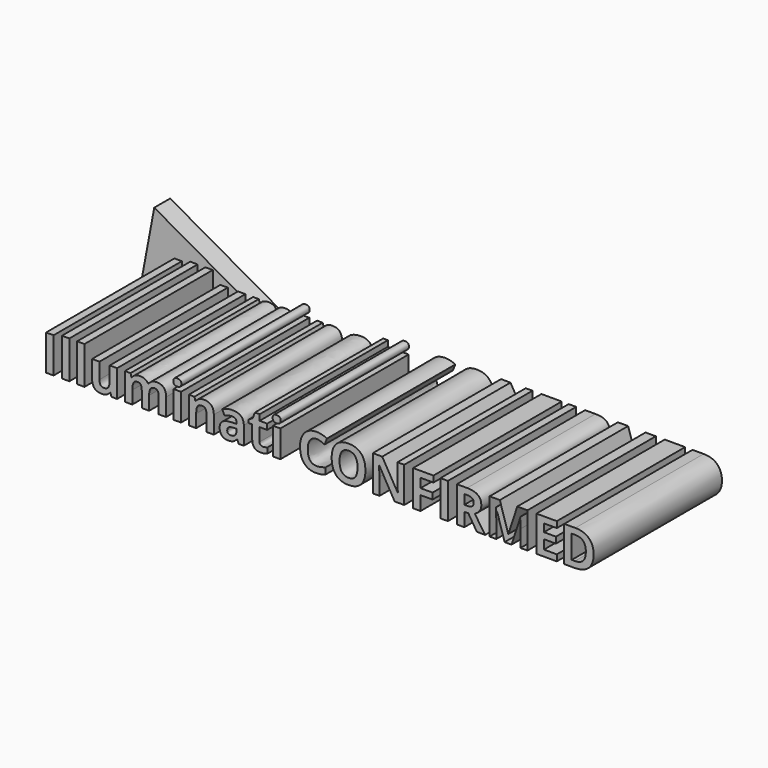
from build123d import *

# Parameters (mm, degrees)
F1_DEPTH     = 3.1
F3_TEXT_SIZE = 7.7416809897
F4_DEPTH     = 25


# Not quite as in the source:
# - Text() gives the source's letters only with a copy of the font that has no kerning and outlines rounded to 1/6400 em; it was checked with that copy


with BuildPart() as f1:
    # F0 (on Front) → F1 (new body)
    with BuildSketch(Plane.XZ):
        Polygon((4.9203070812, 26.2575037777), (0, 0), (22.8598080575, 16.1059461534), align=None)
    extrude(amount=F1_DEPTH)

    # F3 (on face) → F4 (join)
    with BuildSketch(Plane.XZ.offset(3.1)):
        with Locations((7.358269766, 14.7775895894)):
            Text('Illuminati CONFIRMED', F3_TEXT_SIZE, font='Open Sans', font_style=FontStyle.BOLD, text_align=(TextAlign.LEFT, TextAlign.BOTTOM))
    extrude(amount=F4_DEPTH)


solid = f1.part
